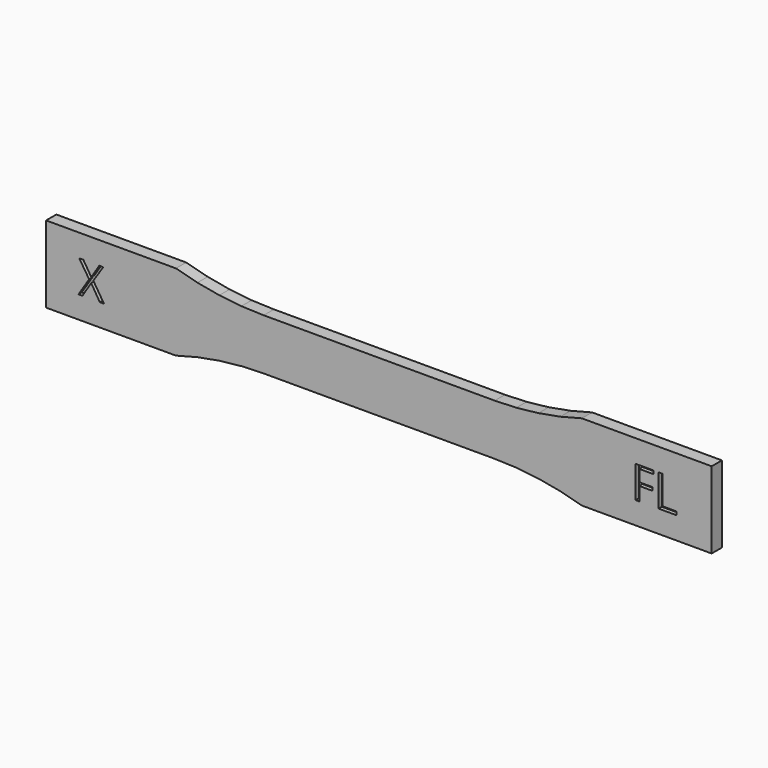
from build123d import *

# Parameters (mm, degrees)
F1_DEPTH     = 3.18
F2_TEXT_SIZE = 11.1111111111
F3_DEPTH     = 1


# Not quite as in the source:
# - Text() gives the source's letters only with a copy of the font that has no kerning and outlines rounded to 1/6400 em; it was checked with that copy


with BuildPart() as f1:
    # F0 (on Front) → F1 (new body)
    with BuildSketch(Plane.XZ):
        Polygon((-50.34, -9.525), (-45.165, -8.175), (-45, -8.13), (-39.57, -7.14), (-34.26, -6.57), (-34.095, -6.54), (-28.57501, -6.345), (28.575, -6.345), (34.095, -6.54), (39.56999, -7.14), (45, -8.13), (50.34, -9.525), (82.545, -9.525), (82.545, 9.525), (50.34, 9.525), (45, 8.145), (39.56999, 7.155), (34.095, 6.555), (28.73999, 6.36), (-28.57501, 6.36), (-34.095, 6.555), (-39.57, 7.155), (-45, 8.145), (-50.34, 9.525), (-82.545, 9.525), (-82.545, -9.525), align=None)
    extrude(amount=F1_DEPTH)

    # F2 (on face) → F3 (cut)
    with BuildSketch(Plane.XZ.offset(3.18)):
        with Locations((-74.545, -4)):
            Text('X', F2_TEXT_SIZE, font='Open Sans', text_align=(TextAlign.LEFT, TextAlign.BOTTOM))
        with Locations((62.5779861111, -4)):
            Text('FL', F2_TEXT_SIZE, font='Open Sans', text_align=(TextAlign.LEFT, TextAlign.BOTTOM))
    extrude(amount=-F3_DEPTH, mode=Mode.SUBTRACT)


solid = f1.part
